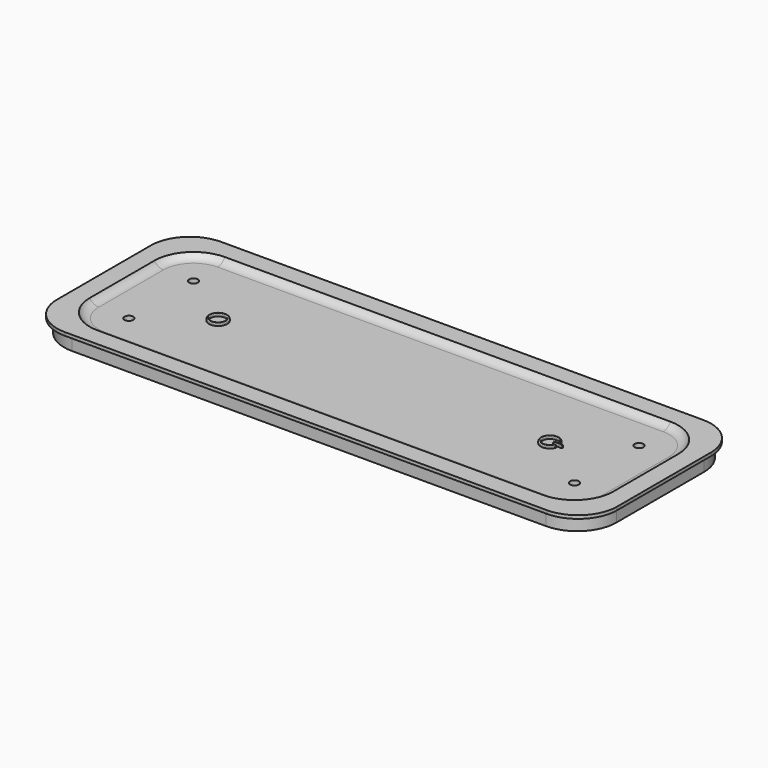
from build123d import *

# Parameters (mm, degrees)
F0_W          = 215
F0_H          = 75
F1_DEPTH      = 1.25
F2_R          = 15
F3_W          = 212
F3_H          = 72
F4_DEPTH      = 5.25
F5_T1_DEPTH   = 42.75
F7_W          = 201
F7_H          = 61
F8_DEPTH      = 2
F9_R          = 15
F10_T1_DEPTH  = 31
F10_T3_DEPTH  = 171
F10_T6_ANGLE  = 90
F10_T8_ANGLE  = 90
F10_T10_ANGLE = 90
F10_T12_ANGLE = 90
F11_W         = 45.625
F11_H         = 3.75
F12_DEPTH     = 12
F13_W         = 153
F13_H         = 55
F14_DEPTH     = 4
F16_D         = 3.4
F17_R         = 3.5
F17_R_2       = 2.75
F17_W         = 3.5
F17_H         = 0.75
F18_DEPTH     = 1.5
F19_R         = 0.37499


# Not quite as in the source:
# - a fillet or chamfer that OpenCascade refuses, or shapes differently, is made with other operations: its cross-section is extruded or revolved along the edge and cut away or added
# - a fillet or chamfer is up to 0.001 mm smaller than in the source, because OpenCascade refuses the exact size


with BuildPart() as f1:
    # F0 (on Top) → F1 (new body)
    with BuildSketch(Plane.XY):
        Rectangle(F0_W, F0_H)
    extrude(amount=F1_DEPTH)

    # F2
    f2_edges = [f1.edges().sort_by_distance(p)[0] for p in [
        (107.5, -37.5, 0.625),
        (107.5, 37.5, 0.625),
        (-107.5, 37.5, 0.625),
        (-107.5, -37.5, 0.625),
    ]]
    fillet(f2_edges, radius=F2_R)

    # F3 (on face) → F4 (join)
    with BuildSketch(Plane(origin=(0, 0, 0), x_dir=(1, 0, 0), z_dir=(0, 0, -1))):
        Rectangle(F3_W, F3_H)
    extrude(amount=F4_DEPTH)

    # F5: fillet of radius 15 on 4 edges, made by hand

    # F5_s2 → F5_t1 (cut)
    with BuildSketch(Plane.XY.offset(-42.75)):
        with BuildLine():
            ThreePointArc((-106, -21), (-101.6066017178, -31.6066017178), (-91, -36))
            Line((-91, -36), (-106, -36))
            Line((-106, -36), (-106, -21))
        make_face()
        with BuildLine():
            ThreePointArc((-91, 36), (-101.6066017178, 31.6066017178), (-106, 21))
            Line((-106, 21), (-106, 36))
            Line((-106, 36), (-91, 36))
        make_face()
        with BuildLine():
            ThreePointArc((91, 36), (101.6066017178, 31.6066017178), (106, 21))
            Line((106, 21), (106, 36))
            Line((106, 36), (91, 36))
        make_face()
        with BuildLine():
            ThreePointArc((106, -21), (101.6066017178, -31.6066017178), (91, -36))
            Line((91, -36), (106, -36))
            Line((106, -36), (106, -21))
        make_face()
    extrude(amount=F5_T1_DEPTH, mode=Mode.SUBTRACT)

    # F7 (on face) → F8 (cut)
    with BuildSketch(Plane.XY.offset(1.25)):
        Rectangle(F7_W, F7_H)
    extrude(amount=-F8_DEPTH, mode=Mode.SUBTRACT)

    # F9
    f9_edges = [f1.edges().sort_by_distance(p)[0] for p in [
        (-100.5, 30.5, 0.25),
        (-100.5, -30.5, 0.25),
        (100.5, 30.5, 0.25),
        (100.5, -30.5, 0.25),
    ]]
    fillet(f9_edges, radius=F9_R)

    # F10: fillet of radius 4 on 1 edges, made by hand

    # F10_s2 → F10_t1 (join)
    with BuildSketch(Plane.XZ.offset(-15.5)):
        with BuildLine():
            ThreePointArc((-100.5, 1.25), (-99.0358983849, -0.2141016151), (-97.0358983849, -0.75))
            Line((-97.0358983849, -0.75), (-100.5, -0.75))
            Line((-100.5, -0.75), (-100.5, 1.25))
        make_face()
        with BuildLine():
            ThreePointArc((100.5, 1.25), (99.0358983849, -0.2141016151), (97.0358983849, -0.75))
            Line((97.0358983849, -0.75), (100.5, -0.75))
            Line((100.5, -0.75), (100.5, 1.25))
        make_face()
    extrude(amount=F10_T1_DEPTH)

    # F10_s4 → F10_t3 (join)
    with BuildSketch(Plane.YZ.offset(-85.5)):
        with BuildLine():
            ThreePointArc((-30.5, 1.25), (-29.0358983849, -0.2141016151), (-27.0358983849, -0.75))
            Line((-27.0358983849, -0.75), (-30.5, -0.75))
            Line((-30.5, -0.75), (-30.5, 1.25))
        make_face()
        with BuildLine():
            ThreePointArc((30.5, 1.25), (29.0358983849, -0.2141016151), (27.0358983849, -0.75))
            Line((27.0358983849, -0.75), (30.5, -0.75))
            Line((30.5, -0.75), (30.5, 1.25))
        make_face()
    extrude(amount=F10_T3_DEPTH)

    # F10_s5 → F10_t6 (revolve)
    with BuildSketch(Plane.YZ.offset(-85.5)):
        with BuildLine():
            ThreePointArc((30.5, 1.25), (29.0358983849, -0.2141016151), (27.0358983849, -0.75))
            Line((27.0358983849, -0.75), (30.5, -0.75))
            Line((30.5, -0.75), (30.5, 1.25))
        make_face()
    revolve(axis=Axis((-85.5, 15.5, -0.75), (0, 0, 1)), revolution_arc=F10_T6_ANGLE)

    # F10_s7 → F10_t8 (revolve)
    with BuildSketch(Plane.XZ.offset(15.5)):
        with BuildLine():
            ThreePointArc((-100.5, 1.25), (-99.0358983849, -0.2141016151), (-97.0358983849, -0.75))
            Line((-97.0358983849, -0.75), (-100.5, -0.75))
            Line((-100.5, -0.75), (-100.5, 1.25))
        make_face()
    revolve(axis=Axis((-85.5, -15.5, -0.75), (0, 0, 1)), revolution_arc=F10_T8_ANGLE)

    # F10_s9 → F10_t10 (revolve)
    with BuildSketch(Plane.YZ.offset(85.5)):
        with BuildLine():
            ThreePointArc((-30.5, 1.25), (-29.0358983849, -0.2141016151), (-27.0358983849, -0.75))
            Line((-27.0358983849, -0.75), (-30.5, -0.75))
            Line((-30.5, -0.75), (-30.5, 1.25))
        make_face()
    revolve(axis=Axis((85.5, -15.5, -0.75), (0, 0, 1)), revolution_arc=F10_T10_ANGLE)

    # F10_s11 → F10_t12 (revolve)
    with BuildSketch(Plane.YZ.offset(85.5)):
        with BuildLine():
            ThreePointArc((30.5, 1.25), (29.0358983849, -0.2141016151), (27.0358983849, -0.75))
            Line((27.0358983849, -0.75), (30.5, -0.75))
            Line((30.5, -0.75), (30.5, 1.25))
        make_face()
    revolve(axis=Axis((85.5, 15.5, -0.75), (0, 0, -1)), revolution_arc=F10_T12_ANGLE)

    # F11 (on face) → F12 (cut)
    with BuildSketch(Plane(origin=(0, 36, 0), x_dir=(-1, 0, 0), z_dir=(0, 1, 0))):
        with Locations((-53.6875, -3.375)):
            Rectangle(F11_W, F11_H)
        with Locations((53.6875, -3.375)):
            Rectangle(F11_W, F11_H)
    extrude(amount=-F12_DEPTH, mode=Mode.SUBTRACT)

    # F13 (on face) → F14 (cut)
    with BuildSketch(Plane(origin=(0, 0, -5.25), x_dir=(1, 0, 0), z_dir=(0, 0, -1))):
        with Locations((0, 6)):
            Rectangle(F13_W, F13_H)
    extrude(amount=-F14_DEPTH, mode=Mode.SUBTRACT)

    # F16 (through all)
    with Locations(Plane.XY.offset(1.25)):
        with Locations((-85.5, 15.5), (-85.5, -15.5), (85.5, 15.5), (85.5, -15.5)):
            Hole(F16_D / 2)

    # F17 (on face) → F18 (join)
    with BuildSketch(Plane(origin=(0, 0, -1.25), x_dir=(1, 0, 0), z_dir=(0, 0, -1))):
        with Locations((-63.6638983849, 0)):
            Circle(F17_R)
        with Locations((-63.6638983849, 0)):
            Circle(F17_R_2, mode=Mode.SUBTRACT)
        with BuildLine():
            Line((66.2986806863, 0.7876688543), (67.0194815177, 0.9950185116))
            ThreePointArc((67.0194815177, 0.9950185116), (60.1639068064, -0.0076779243), (67.0238147407, -0.9802867343))
            Line((67.0238147407, -0.9802867343), (66.2986806863, -0.7876688543))
            ThreePointArc((66.2986806863, -0.7876688543), (60.9138983849, 0), (66.2986806863, 0.7876688543))
        make_face()
        with Locations((66.7888983849, 0)):
            Rectangle(F17_W, F17_H)
    extrude(amount=-F18_DEPTH)

    # F19 (radius 0.375 in the source; OpenCascade refuses exactly that, so slightly less here)
    f19_edges = [f1.edges().sort_by_distance(p)[0] for p in [
        (-66.413898, 0, 0.25),
        (-67.163898, 0, 0.25),
        (60.913898, 0, 0.25),
        (60.163907, 0.007678, 0.25),
        (67.019482, -0.995019, -0.25),
        (66.659081, -0.891344, 0.25),
        (66.298681, -0.787669, -0.25),
        (66.661248, 0.883978, 0.25),
        (66.298681, 0.787669, -0.25),
        (67.023815, 0.980287, -0.25),
        (65.038898, 0, 0.25),
        (65.038898, -0.375, -0.25),
        (65.038898, 0.375, -0.25),
        (66.788898, -0.375, 0.25),
        (66.788898, 0.375, 0.25),
        (68.538898, -0.375, -0.25),
        (68.538898, 0.375, -0.25),
        (68.538898, 0, 0.25),
    ]]
    fillet(f19_edges, radius=F19_R)


solid = f1.part
